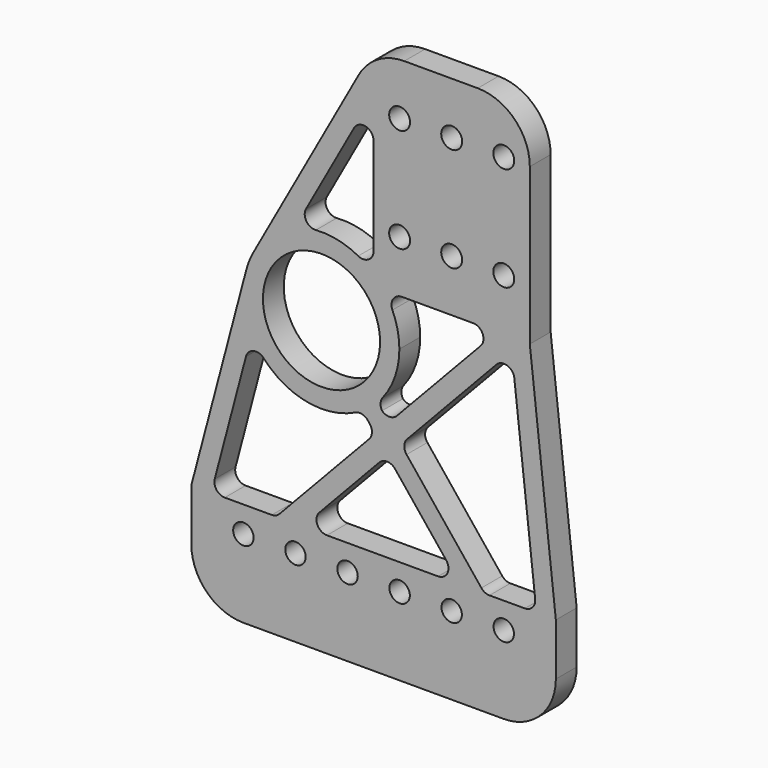
from build123d import *

# Parameters (mm, degrees)
F0_R        = 14.2875
F0_R_2      = 2.4892
F0_R_3      = 2.5527
F1_DEPTH    = 6.35
F2_R        = 12.7
F3_T1_DEPTH = 6.35


# Not quite as in the source:
# - a fillet or chamfer that OpenCascade refuses, or shapes differently, is made with other operations: its cross-section is extruded or revolved along the edge and cut away or added


with BuildPart() as f1:
    # F0 (on Front) → F1 (new body)
    with BuildSketch(Plane.XZ):
        with BuildLine():
            ThreePointArc((-73.767427816, -72.0958683029), (-74.7686667008, -74.2040007111), (-75.5037002278, -76.4190463696))
            ThreePointArc((-75.5037002278, -76.4190463696), (-76.040577327, -83.1861139792), (-74.1626528233, -89.7095211112))
            ThreePointArc((-74.1626528233, -89.7095211112), (-62.3780093009, -99.5325368374), (-47.1798914821, -97.4380976105))
            ThreePointArc((-47.1798914821, -97.4380976105), (-45.257025222, -96.0801463905), (-43.5169789975, -94.4946857926))
            ThreePointArc((-43.5169789975, -94.4946857926), (-39.5526914627, -88.4089490455), (-38.1635, -81.28))
            ThreePointArc((-38.1635, -81.28), (-39.1453760307, -75.2533344231), (-41.9894498038, -69.85))
            Line((-41.9894498038, -69.85), (-44.1945328452, -69.85))
            Line((-44.1945328452, -69.85), (-44.45, -69.85))
            Line((-44.45, -69.85), (-44.45, -67.1662768112))
            ThreePointArc((-44.45, -67.1662768112), (-45.5081692727, -66.2815014229), (-46.6277808452, -65.4758838808))
            ThreePointArc((-46.6277808452, -65.4758838808), (-54.8730151863, -62.430529917), (-63.6062431678, -63.4249137104))
            ThreePointArc((-63.6062431678, -63.4249137104), (-69.474566384, -66.8372770678), (-73.767427816, -72.0958683029))
        make_face()
        with Locations((-57.15, -81.28)):
            Circle(F0_R, mode=Mode.SUBTRACT)
        with BuildLine():
            Line((-44.45, -28.7643166542), (-44.45, -19.05))
            Line((-44.45, -19.05), (-73.767427816, -72.0958683029))
            ThreePointArc((-73.767427816, -72.0958683029), (-69.474566384, -66.8372770678), (-63.6062431678, -63.4249137104))
            Line((-63.6062431678, -63.4249137104), (-44.45, -28.7643166542))
        make_face()
        with BuildLine():
            Line((-75.5037002278, -76.4190463696), (-88.9, -127))
            Line((-88.9, -127), (-84.0389876487, -127))
            Line((-84.0389876487, -127), (-74.1626528233, -89.7095211112))
            ThreePointArc((-74.1626528233, -89.7095211112), (-76.040577327, -83.1861139792), (-75.5037002278, -76.4190463696))
        make_face()
        Polygon((-84.0389876487, -127), (-88.9, -127), (-88.9, -152.4), (0, -152.4), (0, -127), (-4.727917196, -127), (-17.3966372237, -127), (-23.4247913477, -127), (-61.7257976966, -127), (-68.1836898087, -127), align=None)
        with Locations((-76.2, -133.35)):
            Circle(F0_R_2, mode=Mode.SUBTRACT)
        with Locations((-63.5, -133.35)):
            Circle(F0_R_2, mode=Mode.SUBTRACT)
        with Locations((-50.8, -133.35)):
            Circle(F0_R_2, mode=Mode.SUBTRACT)
        with Locations((-38.1, -133.35)):
            Circle(F0_R_2, mode=Mode.SUBTRACT)
        with Locations((-25.4, -133.35)):
            Circle(F0_R_2, mode=Mode.SUBTRACT)
        with Locations((-12.7, -133.35)):
            Circle(F0_R_2, mode=Mode.SUBTRACT)
        Polygon((-4.727917196, -127), (0, -127), (-6.35, -69.85), (-11.077917196, -69.85), (-10.7374740973, -72.913987888), align=None)
        with BuildLine():
            Line((-6.35, -69.85), (-6.35, -19.05))
            Line((-6.35, -19.05), (-44.45, -19.05))
            Line((-44.45, -19.05), (-44.45, -28.7643166542))
            Line((-44.45, -28.7643166542), (-44.45, -62.9496581004))
            Line((-44.45, -62.9496581004), (-44.45, -67.1662768112))
            ThreePointArc((-44.45, -67.1662768112), (-43.7416474883, -67.8374085396), (-43.0687114356, -68.5440471649))
            ThreePointArc((-43.0687114356, -68.5440471649), (-42.5145067823, -69.1849795153), (-41.9894498038, -69.85))
            Line((-41.9894498038, -69.85), (-14.3068632521, -69.85))
            Line((-14.3068632521, -69.85), (-11.077917196, -69.85))
            Line((-11.077917196, -69.85), (-6.35, -69.85))
        make_face()
        with Locations((-38.1, -57.15)):
            Circle(F0_R_3, mode=Mode.SUBTRACT)
        with Locations((-25.4, -57.15)):
            Circle(F0_R_3, mode=Mode.SUBTRACT)
        with Locations((-12.7, -57.15)):
            Circle(F0_R_3, mode=Mode.SUBTRACT)
        with Locations((-38.1, -31.75)):
            Circle(F0_R_3, mode=Mode.SUBTRACT)
        with Locations((-25.4, -31.75)):
            Circle(F0_R_3, mode=Mode.SUBTRACT)
        with Locations((-12.7, -31.75)):
            Circle(F0_R_3, mode=Mode.SUBTRACT)
        Polygon((-44.0209157758, -101.3692673783), (-68.1836898087, -127), (-61.7257976966, -127), (-41.0492709397, -105.0673142856), align=None)
        Polygon((-40.7666595063, -97.9173056039), (-44.0209157758, -101.3692673783), (-41.0492709397, -105.0673142856), (-37.7950146701, -101.6153525111), align=None)
        Polygon((-10.7374740973, -72.913987888), (-11.077917196, -69.85), (-14.3068632521, -69.85), (-40.7666595063, -97.9173056039), (-37.7950146701, -101.6153525111), align=None)
        with BuildLine():
            Line((-47.1798914821, -97.4380976105), (-44.0209157758, -101.3692673783))
            Line((-44.0209157758, -101.3692673783), (-40.7666595063, -97.9173056039))
            Line((-40.7666595063, -97.9173056039), (-43.5169789975, -94.4946857926))
            ThreePointArc((-43.5169789975, -94.4946857926), (-45.257025222, -96.0801463905), (-47.1798914821, -97.4380976105))
        make_face()
        Polygon((-23.4247913477, -127), (-17.3966372237, -127), (-37.7950146701, -101.6153525111), (-41.0492709397, -105.0673142856), align=None)
        with BuildLine():
            ThreePointArc((-43.0687114356, -68.5440471649), (-43.7416474883, -67.8374085396), (-44.45, -67.1662768112))
            Line((-44.45, -67.1662768112), (-44.45, -69.85))
            Line((-44.45, -69.85), (-44.1945328452, -69.85))
            Line((-44.1945328452, -69.85), (-43.0687114356, -68.5440471649))
        make_face()
        with BuildLine():
            Line((-44.1945328452, -69.85), (-41.9894498038, -69.85))
            ThreePointArc((-41.9894498038, -69.85), (-42.5145067823, -69.1849795153), (-43.0687114356, -68.5440471649))
            Line((-43.0687114356, -68.5440471649), (-44.1945328452, -69.85))
        make_face()
    extrude(amount=F1_DEPTH)

    # F2
    f2_edges = [f1.edges().sort_by_distance(p)[0] for p in [
        (-6.35, -3.175, -19.05),
        (-88.9, -3.175, -152.4),
        (0, -3.175, -152.4),
        (-44.45, -3.175, -19.05),
    ]]
    fillet(f2_edges, radius=F2_R)

    # F3: fillet of radius 2.54 on 21 edges, made by hand

    # F3_s2 → F3_t1 (join)
    with BuildSketch(Plane.XZ):
        with BuildLine():
            ThreePointArc((-58.5225193342, -62.3431741591), (-60.8457611864, -61.1786129184), (-60.9292012272, -58.5811731507))
            Line((-60.9292012272, -58.5811731507), (-63.6062431678, -63.4249137104))
            ThreePointArc((-63.6062431678, -63.4249137104), (-61.1015719267, -62.7092633006), (-58.5225193342, -62.3431741591))
        make_face()
        with BuildLine():
            ThreePointArc((-42.2061934884, -92.9919524074), (-42.7469750096, -94.5742269942), (-42.1869747431, -96.1498021981))
            Line((-42.1869747431, -96.1498021981), (-43.5169789975, -94.4946857926))
            ThreePointArc((-43.5169789975, -94.4946857926), (-42.8418442978, -93.7605393574), (-42.2061934884, -92.9919524074))
        make_face()
        with BuildLine():
            ThreePointArc((-48.929563825, -98.3946607137), (-47.2679726242, -98.2071715059), (-45.8498872277, -99.0932140161))
            Line((-45.8498872277, -99.0932140161), (-47.1798914821, -97.4380976105))
            ThreePointArc((-47.1798914821, -97.4380976105), (-48.0421609425, -97.9393652326), (-48.929563825, -98.3946607137))
        make_face()
        with BuildLine():
            ThreePointArc((-71.2393441045, -94.007040699), (-73.7227097824, -93.2411748511), (-75.5795507042, -95.0593600393))
            Line((-75.5795507042, -95.0593600393), (-74.1626528233, -89.7095211112))
            ThreePointArc((-74.1626528233, -89.7095211112), (-72.8487490545, -91.958785529), (-71.2393441045, -94.007040699))
        make_face()
        with BuildLine():
            ThreePointArc((-44.45, -38.6110805765), (-46.35556752, -36.1515896884), (-49.2130672664, -37.3824341956))
            Line((-49.2130672664, -37.3824341956), (-44.45, -28.7643166542))
            Line((-44.45, -28.7643166542), (-44.45, -38.6110805765))
        make_face()
        with BuildLine():
            ThreePointArc((-38.7656990781, -95.7947810274), (-40.7142143439, -96.5904542384), (-42.5938492637, -95.6434694613))
            Line((-42.5938492637, -95.6434694613), (-40.7666595063, -97.9173056039))
            Line((-40.7666595063, -97.9173056039), (-38.7656990781, -95.7947810274))
        make_face()
        with BuildLine():
            ThreePointArc((-67.4317191857, -126.2023449812), (-68.2734267993, -126.7920759263), (-69.2799166769, -127))
            Line((-69.2799166769, -127), (-68.1836898087, -127))
            Line((-68.1836898087, -127), (-67.4317191857, -126.2023449812))
        make_face()
        with BuildLine():
            ThreePointArc((-80.7386977088, -127), (-82.7515748526, -126.0091693271), (-83.1940422209, -123.8097051999))
            Line((-83.1940422209, -123.8097051999), (-84.0389876487, -127))
            Line((-84.0389876487, -127), (-80.7386977088, -127))
        make_face()
        with BuildLine():
            ThreePointArc((-20.1921413698, -69.85), (-17.8600654435, -71.3835101223), (-18.3439438786, -74.1323449812))
            Line((-18.3439438786, -74.1323449812), (-14.3068632521, -69.85))
            Line((-14.3068632521, -69.85), (-20.1921413698, -69.85))
        make_face()
        with BuildLine():
            ThreePointArc((-45.4063150305, -99.6452149726), (-44.8482495326, -101.3365661623), (-45.5380702337, -102.9785933689))
            Line((-45.5380702337, -102.9785933689), (-44.0209157758, -101.3692673783))
            Line((-44.0209157758, -101.3692673783), (-45.4063150305, -99.6452149726))
        make_face()
        with BuildLine():
            ThreePointArc((-43.0502313678, -107.1898388621), (-41.1017161021, -106.394165651), (-39.2220811823, -107.3411504281))
            Line((-39.2220811823, -107.3411504281), (-41.0492709397, -105.0673142856))
            Line((-41.0492709397, -105.0673142856), (-43.0502313678, -107.1898388621))
        make_face()
        with BuildLine():
            ThreePointArc((-36.2778602123, -100.0060265206), (-36.9676809133, -101.6480537272), (-36.4096154155, -103.3394049169))
            Line((-36.4096154155, -103.3394049169), (-37.7950146701, -101.6153525111))
            Line((-37.7950146701, -101.6153525111), (-36.2778602123, -100.0060265206))
        make_face()
        with BuildLine():
            ThreePointArc((-57.68871707, -122.7176550188), (-58.1725955051, -125.4664898777), (-55.8405195788, -127))
            Line((-55.8405195788, -127), (-61.7257976966, -127))
            Line((-61.7257976966, -127), (-57.68871707, -122.7176550188))
        make_face()
        with BuildLine():
            ThreePointArc((-26.7443717706, -122.8689665849), (-26.4338196217, -125.5578103492), (-28.724324465, -127))
            Line((-28.724324465, -127), (-23.4247913477, -127))
            Line((-23.4247913477, -127), (-26.7443717706, -122.8689665849))
        make_face()
        with BuildLine():
            ThreePointArc((-5.0413056489, -124.1795039238), (-5.6731451696, -126.1539805144), (-7.565770335, -127))
            Line((-7.565770335, -127), (-4.727917196, -127))
            Line((-4.727917196, -127), (-5.0413056489, -124.1795039238))
        make_face()
        with BuildLine():
            ThreePointArc((-14.5038036224, -76.9091328532), (-11.8502584516, -76.2425330207), (-10.1311414451, -78.3709817581))
            Line((-10.1311414451, -78.3709817581), (-10.7374740973, -72.913987888))
            Line((-10.7374740973, -72.913987888), (-14.5038036224, -76.9091328532))
        make_face()
        with BuildLine():
            ThreePointArc((-16.1792469636, -127), (-17.2770573128, -126.7505048433), (-18.159199658, -126.0510334151))
            Line((-18.159199658, -126.0510334151), (-17.3966372237, -127))
            Line((-17.3966372237, -127), (-16.1792469636, -127))
        make_face()
        with BuildLine():
            ThreePointArc((-39.8582276098, -73.4389675516), (-39.6798917034, -71.0139145341), (-37.5449470225, -69.85))
            Line((-37.5449470225, -69.85), (-41.9894498038, -69.85))
            ThreePointArc((-41.9894498038, -69.85), (-40.8249124862, -71.5857388153), (-39.8582276098, -73.4389675516))
        make_face()
        with BuildLine():
            ThreePointArc((-44.45, -62.3019968846), (-45.6848952053, -64.4810566531), (-48.188820059, -64.5412892876))
            ThreePointArc((-48.188820059, -64.5412892876), (-46.2401732835, -65.7409246328), (-44.45, -67.1662768112))
            Line((-44.45, -67.1662768112), (-44.45, -62.3019968846))
        make_face()
    extrude(amount=F3_T1_DEPTH)


solid = f1.part
